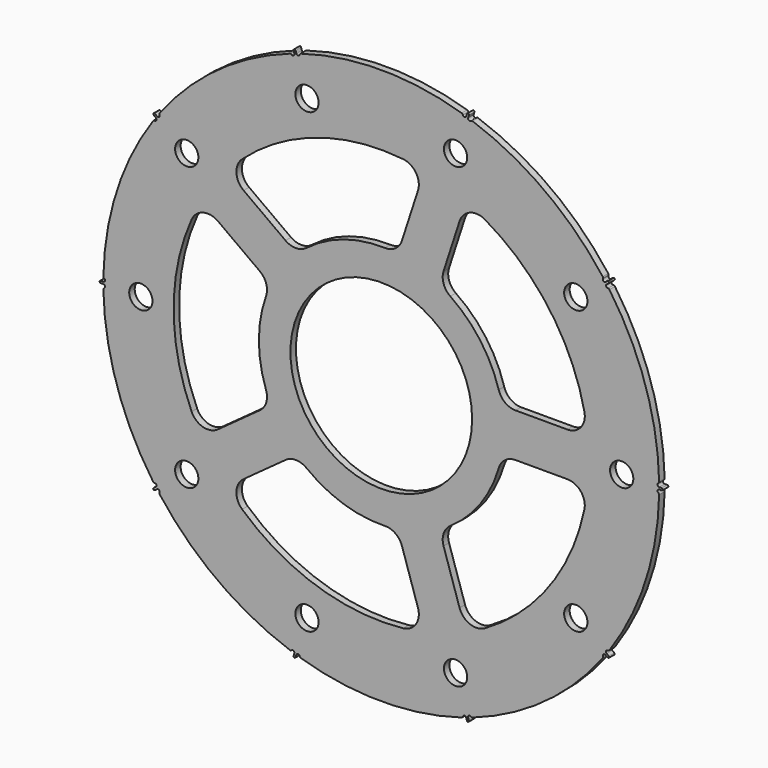
from build123d import *

# Parameters (mm, degrees)
F1_DEPTH        = 2
F2_R            = 26.391
F3_DEPTH        = 2
F4_D            = 6.7564
F6_DEPTH        = 2
F6_COPIES_COUNT = 5
F7_R            = 5.08


# Not quite as in the source:
# - a pattern or mirror of a feature is missing from the dataset's text; its kind, count and spacing are read off the source's solid


with BuildPart() as f1:
    # F0 (on Front) → F1 (new body)
    with BuildSketch(Plane.XZ):
        with BuildLine():
            ThreePointArc((23.7036118773, 76.9298434376), (23.5816837061, 77.1596187003), (23.3608317089, 77.2970506673))
            ThreePointArc((23.3608317089, 77.2970506673), (-0.0001147149, 80.75), (-23.361051328, 77.2969842934))
            ThreePointArc((-23.361051328, 77.2969842934), (-23.5811818782, 77.1603225108), (-23.7033557347, 76.9318330127))
            ThreePointArc((-23.7033557347, 76.9318330127), (-24.1707219857, 76.5456761593), (-24.6669025773, 76.8940339476))
            Line((-24.6669025773, 76.8940339476), (-24.8986653231, 77.6073263348))
            ThreePointArc((-24.8986653231, 77.6073263348), (-25.2766873763, 77.7999381914), (-25.4692992328, 77.4219161382))
            Line((-25.4692992328, 77.4219161382), (-25.237536487, 76.7086237509))
            ThreePointArc((-25.237536487, 76.7086237509), (-25.4350730727, 76.1345635963), (-26.0408720416, 76.174229364))
            ThreePointArc((-26.0408720416, 76.174229364), (-26.2745725149, 76.2884538755), (-26.5340260173, 76.2698251255))
            ThreePointArc((-26.5340260173, 76.2698251255), (-47.4630213735, 65.3321000288), (-64.3327843897, 48.8073376194))
            ThreePointArc((-64.3327843897, 48.8073376194), (-64.4305459654, 48.5673864238), (-64.3950839344, 48.3107225458))
            ThreePointArc((-64.3950839344, 48.3107225458), (-64.5462138705, 47.7236040991), (-65.1523919718, 47.7137838357))
            Line((-65.1523919718, 47.7137838357), (-65.7591547176, 48.154622775))
            ThreePointArc((-65.7591547176, 48.154622775), (-66.1781953916, 48.0882532523), (-66.111825869, 47.6692125783))
            Line((-66.111825869, 47.6692125783), (-65.5050631232, 47.2283736391))
            ThreePointArc((-65.5050631232, 47.2283736391), (-65.3274494852, 46.6478401264), (-65.8408660995, 46.3238507067))
            ThreePointArc((-65.8408660995, 46.3238507067), (-66.0970732373, 46.2788945861), (-66.2960258255, 46.1113206684))
            ThreePointArc((-66.2960258255, 46.1113206684), (-76.7989052383, 24.9607603697), (-80.7338185677, 1.6761488419))
            ThreePointArc((-80.7338185677, 1.6761488419), (-80.6718695698, 1.4245614344), (-80.4923169417, 1.2377600541))
            ThreePointArc((-80.4923169417, 1.2377600541), (-80.2694840641, 0.6739393053), (-80.7541202437, 0.3096919972))
            Line((-80.7541202437, 0.3096919972), (-81.5041202437, 0.3096919972))
            ThreePointArc((-81.5041202437, 0.3096919972), (-81.8041202437, 0.0096919972), (-81.5041202437, -0.2903080028))
            Line((-81.5041202437, -0.2903080028), (-80.7541202437, -0.2903080028))
            ThreePointArc((-80.7541202437, -0.2903080028), (-80.2691987549, -0.6555708034), (-80.4941253183, -1.219462464))
            ThreePointArc((-80.4941253183, -1.219462464), (-80.6749767021, -1.4064275067), (-80.7374352495, -1.6589390512))
            ThreePointArc((-80.7374352495, -1.6589390512), (-76.8024557631, -24.9435393989), (-66.2995162565, -46.0940698564))
            ThreePointArc((-66.2995162565, -46.0940698564), (-66.1015190967, -46.2611956373), (-65.8464588727, -46.3067827417))
            ThreePointArc((-65.8464588727, -46.3067827417), (-65.3347777668, -46.63194543), (-65.5127574763, -47.2114896916))
            Line((-65.5127574763, -47.2114896916), (-66.119520222, -47.6523286308))
            ThreePointArc((-66.119520222, -47.6523286308), (-66.1858897447, -48.0713693048), (-65.7668490707, -48.1377388274))
            Line((-65.7668490707, -48.1377388274), (-65.1600863249, -47.6968998882))
            ThreePointArc((-65.1600863249, -47.6968998882), (-64.5530805121, -47.7073740016), (-64.4036027223, -48.2957804549))
            ThreePointArc((-64.4036027223, -48.2957804549), (-64.4400192705, -48.5533401281), (-64.342126735, -48.7943384719))
            ThreePointArc((-64.342126735, -48.7943384719), (-47.472316768, -65.3190529502), (-26.5432903353, -76.2567185827))
            ThreePointArc((-26.5432903353, -76.2567185827), (-26.2848731988, -76.275546369), (-26.0517297154, -76.1625064731))
            ThreePointArc((-26.0517297154, -76.1625064731), (-25.4466451721, -76.124810006), (-25.2499862118, -76.698285011))
            Line((-25.2499862118, -76.698285011), (-25.4817489576, -77.4115773982))
            ThreePointArc((-25.4817489576, -77.4115773982), (-25.289137101, -77.7895994514), (-24.9111150478, -77.5969875949))
            Line((-24.9111150478, -77.5969875949), (-24.679352302, -76.8836952076))
            ThreePointArc((-24.679352302, -76.8836952076), (-24.1821177544, -76.5353798786), (-23.7153310466, -76.9235498585))
            ThreePointArc((-23.7153310466, -76.9235498585), (-23.5934028755, -77.1533251211), (-23.3725508783, -77.2907570882))
            ThreePointArc((-23.3725508783, -77.2907570882), (-0.0116044544, -80.7437064208), (23.3493321587, -77.2906907142))
            ThreePointArc((23.3493321587, -77.2906907142), (23.5694627088, -77.1540289316), (23.6916365654, -76.9255394336))
            ThreePointArc((23.6916365654, -76.9255394336), (24.1590028164, -76.5393825802), (24.655183408, -76.8877403684))
            Line((24.655183408, -76.8877403684), (24.8869461537, -77.6010327556))
            ThreePointArc((24.8869461537, -77.6010327556), (25.2649682069, -77.7936446122), (25.4575800635, -77.415622559))
            Line((25.4575800635, -77.415622559), (25.2258173177, -76.7023301718))
            ThreePointArc((25.2258173177, -76.7023301718), (25.4233539034, -76.1282700171), (26.0291528723, -76.1679357848))
            ThreePointArc((26.0291528723, -76.1679357848), (26.2628533456, -76.2821602963), (26.522306848, -76.2635315464))
            ThreePointArc((26.522306848, -76.2635315464), (47.4513022041, -65.3258064496), (64.3210652204, -48.8010440403))
            ThreePointArc((64.3210652204, -48.8010440403), (64.4188267961, -48.5610928447), (64.383364765, -48.3044289667))
            ThreePointArc((64.383364765, -48.3044289667), (64.5344947012, -47.71731052), (65.1406728025, -47.7074902566))
            Line((65.1406728025, -47.7074902566), (65.7474355483, -48.1483291958))
            ThreePointArc((65.7474355483, -48.1483291958), (66.1664762223, -48.0819596732), (66.1001066997, -47.6629189992))
            Line((66.1001066997, -47.6629189992), (65.4933439539, -47.22208006))
            ThreePointArc((65.4933439539, -47.22208006), (65.3157303159, -46.6415465472), (65.8291469302, -46.3175571276))
            ThreePointArc((65.8291469302, -46.3175571276), (66.0853540679, -46.272601007), (66.2843066561, -46.1050270893))
            ThreePointArc((66.2843066561, -46.1050270893), (76.787186069, -24.9544667906), (80.7220993984, -1.6698552628))
            ThreePointArc((80.7220993984, -1.6698552628), (80.6601504005, -1.4182678553), (80.4805977724, -1.231466475))
            ThreePointArc((80.4805977724, -1.231466475), (80.2577648948, -0.6676457262), (80.7424010744, -0.3033984181))
            Line((80.7424010744, -0.3033984181), (81.4924010744, -0.3033984181))
            ThreePointArc((81.4924010744, -0.3033984181), (81.7924010744, -0.0033984181), (81.4924010744, 0.2966015819))
            Line((81.4924010744, 0.2966015819), (80.7424010744, 0.2966015819))
            ThreePointArc((80.7424010744, 0.2966015819), (80.2574795855, 0.6618643825), (80.4824061489, 1.2257560431))
            ThreePointArc((80.4824061489, 1.2257560431), (80.6632575328, 1.4127210859), (80.7257160802, 1.6652326303))
            ThreePointArc((80.7257160802, 1.6652326303), (76.7907365938, 24.949832978), (66.2877970872, 46.1003634355))
            ThreePointArc((66.2877970872, 46.1003634355), (66.0897999274, 46.2674892164), (65.8347397034, 46.3130763208))
            ThreePointArc((65.8347397034, 46.3130763208), (65.3230585975, 46.6382390092), (65.5010383069, 47.2177832707))
            Line((65.5010383069, 47.2177832707), (66.1078010527, 47.6586222099))
            ThreePointArc((66.1078010527, 47.6586222099), (66.2275213073, 47.9498138563), (66.0211672681, 48.1876026803))
            ThreePointArc((66.0211672681, 48.1876026803), (65.8829789289, 48.1973831385), (65.7551299013, 48.1440324066))
            Line((65.7551299013, 48.1440324066), (65.1483671556, 47.7031934673))
            ThreePointArc((65.1483671556, 47.7031934673), (64.5413613427, 47.7136675807), (64.391883553, 48.302074034))
            ThreePointArc((64.391883553, 48.302074034), (64.4283001012, 48.5596337072), (64.3304075656, 48.800632051))
            ThreePointArc((64.3304075656, 48.800632051), (47.4605975987, 65.3253465293), (26.5315711659, 76.2630121618))
            ThreePointArc((26.5315711659, 76.2630121618), (26.2731540295, 76.2818399482), (26.040010546, 76.1688000523))
            ThreePointArc((26.040010546, 76.1688000523), (25.4349260028, 76.1311035851), (25.2382670425, 76.7045785902))
            Line((25.2382670425, 76.7045785902), (25.4700297882, 77.4178709774))
            ThreePointArc((25.4700297882, 77.4178709774), (25.2774179317, 77.7958930306), (24.8993958785, 77.603281174))
            Line((24.8993958785, 77.603281174), (24.6676331327, 76.8899887868))
            ThreePointArc((24.6676331327, 76.8899887868), (24.170398585, 76.5416734577), (23.7036118773, 76.9298434376))
        make_face()
    extrude(amount=F1_DEPTH)

    # F2 (on face) → F3 (cut, through all)
    with BuildSketch(Plane.XZ.offset(2)):
        Circle(F2_R)
    extrude(amount=-F3_DEPTH, mode=Mode.SUBTRACT)

    # F4 (through all)
    with Locations(Plane.XZ.offset(2)):
        with Locations((21.5848370571, 66.4312976632), (-21.5848370571, 66.4312976632), (-56.5098370571, 41.0567998726), (-69.85, 0), (-56.5098370571, -41.0567998726), (-21.5848370571, -66.4312976632), (21.5848370571, -66.4312976632), (56.5098370571, -41.0567998726), (69.85, 0), (56.5098370571, 41.0567998726)):
            Hole(F4_D / 2)

    # F5 (on face) → F6 (cut, through all)
    with BuildSketch(Plane.XZ.offset(2)):
        with BuildLine():
            ThreePointArc((12.4986768937, 59.0160037694), (-18.6414501857, 57.3724843455), (-44.8003786791, 40.3984120382))
            Line((-44.8003786791, 40.3984120382), (-24.573808138, 25.7029483444))
            ThreePointArc((-24.573808138, 25.7029483444), (-10.98864432, 33.8195697195), (4.7728144229, 35.2382440324))
            Line((4.7728144229, 35.2382440324), (12.4986768937, 59.0160037694))
        make_face()
    f6 = extrude(amount=-F6_DEPTH, mode=Mode.SUBTRACT)

    # F6_copies: F6 ×5 about axis
    f6_copies_axis = Axis((0, 0, 0), (0, 1, 0))
    for i in range(1, F6_COPIES_COUNT):
        add(f6.rotate(f6_copies_axis, i * 360 / F6_COPIES_COUNT), mode=Mode.SUBTRACT)

    # F7
    f7_edges = [f1.edges().sort_by_distance(p)[0] for p in [
        (-44.800379, -1, 40.398412),
        (-24.573808, -1, 25.702948),
        (4.772814, -1, 35.238244),
        (12.498677, -1, 59.016004),
        (12.498677, -1, -59.016004),
        (4.772814, -1, -35.238244),
        (-44.800379, -1, -40.398412),
        (-24.573808, -1, -25.702948),
        (-52.265251, -1, -30.123896),
        (-32.038681, -1, -15.428433),
        (-32.038681, -1, 15.428433),
        (-52.265251, -1, 30.123896),
        (59.989859, -1, -6.35),
        (34.988442, -1, -6.35),
        (24.577095, -1, -55.091488),
        (16.851232, -1, -31.313728),
        (24.577095, -1, 55.091488),
        (16.851232, -1, 31.313728),
        (59.989859, -1, 6.35),
        (34.988442, -1, 6.35),
    ]]
    fillet(f7_edges, radius=F7_R)


solid = f1.part
